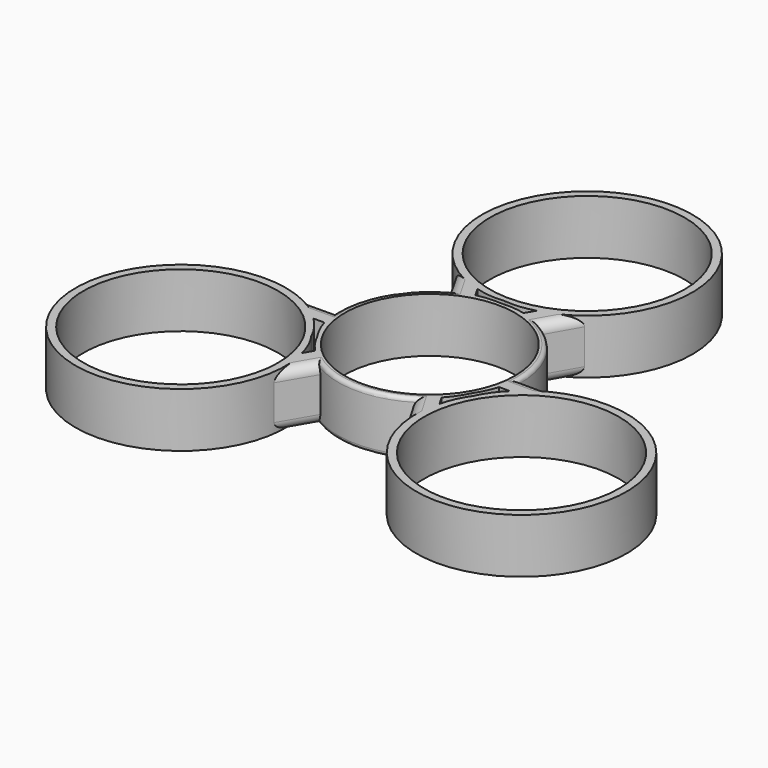
from build123d import *

# Parameters (mm, degrees)
F0_R     = 12.7
F0_R_2   = 11.1125
F1_DEPTH = 7.112
F2_R     = 1.27
F3_R     = 0.50799


# Not quite as in the source:
# - a fillet or chamfer is up to 0.001 mm smaller than in the source, because OpenCascade refuses the exact size
# - ends of sketch curves that miss each other by under 0.0002 mm in the source are joined


with BuildPart() as f1:
    # F0 (on Top) → F1 (new body)
    with BuildSketch(Plane.XY):
        with BuildLine():
            ThreePointArc((8.3638022209, 14.7734709329), (0, 39.3942033225), (-8.3638022209, 14.7734709329))
            Line((-8.3638022209, 14.7734709329), (-5.8662054787, 10.3931058657))
            ThreePointArc((-5.8662054787, 10.3931058657), (-10.3354618297, 5.9671806592), (-11.9337964262, -0.1162717145))
            Line((-11.9337964262, -0.1162717145), (-16.9761022194, -0.1434727603))
            ThreePointArc((-16.9761022194, -0.1434727603), (-34.1163779507, -19.6971066641), (-8.6122978741, -14.6300019249))
            Line((-8.6122978741, -14.6300019249), (-6.0675894575, -10.276836791))
            ThreePointArc((-6.0675894575, -10.276836791), (0, -11.934362834), (6.0675894575, -10.276836791))
            Line((6.0675894575, -10.276836791), (8.6122978741, -14.6300019249))
            ThreePointArc((8.6122978741, -14.6300019249), (34.1163779507, -19.6971066641), (16.9761022194, -0.1434727603))
            Line((16.9761022194, -0.1434727603), (11.9337964262, -0.1162717145))
            ThreePointArc((11.9337964262, -0.1162717145), (10.3354618297, 5.9671806592), (5.8662054787, 10.3931058657))
            Line((5.8662054787, 10.3931058657), (8.3638022209, 14.7734709329))
        make_face()
        with Locations((-22.225, -12.83160756)):
            Circle(F0_R, mode=Mode.SUBTRACT)
        with BuildLine():
            ThreePointArc((-8.9782080284, -9.6422017781), (-9.6052965229, -7.7965006784), (-10.5814479311, -6.109200777))
            ThreePointArc((-10.5814479311, -6.109200777), (-11.5546165578, -4.4201787661), (-12.8394961357, -2.9542534612))
            Line((-12.8394961357, -2.9542534612), (-11.4007424563, -2.9542534612))
            ThreePointArc((-11.4007424563, -2.9542534612), (-10.8372927454, -4.4313928826), (-10.042581953, -5.7980864121))
            ThreePointArc((-10.042581953, -5.7980864121), (-9.2563462346, -7.1696730271), (-8.258831006, -8.3962046475))
            Line((-8.258831006, -8.3962046475), (-8.9782080284, -9.6422017781))
        make_face(mode=Mode.SUBTRACT)
        with Locations((22.225, -12.83160756)):
            Circle(F0_R, mode=Mode.SUBTRACT)
        with BuildLine():
            Line((11.4007424563, -2.9542534612), (12.8394961357, -2.9542534612))
            ThreePointArc((12.8394961357, -2.9542534612), (11.5546165578, -4.4201787661), (10.5814479311, -6.109200777))
            ThreePointArc((10.5814479311, -6.109200777), (9.6052965229, -7.7965006784), (8.9782080284, -9.6422017781))
            Line((8.9782080284, -9.6422017781), (8.258831006, -8.3962046475))
            ThreePointArc((8.258831006, -8.3962046475), (9.2563462346, -7.1696730271), (10.042581953, -5.7980864121))
            ThreePointArc((10.042581953, -5.7980864121), (10.8372927454, -4.4313928826), (11.4007424563, -2.9542534612))
        make_face(mode=Mode.SUBTRACT)
        Circle(F0_R_2, mode=Mode.SUBTRACT)
        with BuildLine():
            ThreePointArc((-3.8612913684, 12.5964559897), (-1.9493229697, 12.2166805672), (-2.6876e-06, 12.2184031057))
            ThreePointArc((-2.6876e-06, 12.2184031057), (1.9493202828, 12.2166814247), (3.8612885145, 12.5964576884))
            Line((3.8612885145, 12.5964576884), (3.1419093526, 11.3504602412))
            ThreePointArc((3.1419093526, 11.3504602412), (1.5809467105, 11.6010677307), (0, 11.5961742969))
            ThreePointArc((0, 11.5961742969), (-1.5809492634, 11.6010670352), (-3.141914346, 11.350458859))
            Line((-3.141914346, 11.350458859), (-3.8612913684, 12.5964559897))
        make_face(mode=Mode.SUBTRACT)
        with Locations((0, 25.6632216382)):
            Circle(F0_R, mode=Mode.SUBTRACT)
    extrude(amount=F1_DEPTH)

    # F2
    f2_edges = [f1.edges().sort_by_distance(p)[0] for p in [
        (-7.339944, -12.453419, 7.112),
        (-14.454949, -0.129872, 7.112),
        (7.339944, -12.453419, 7.112),
        (14.454949, -0.129872, 7.112),
        (7.115004, 12.583288, 7.112),
        (-7.115004, 12.583288, 7.112),
        (-7.339944, -12.453419, 0),
        (7.339944, -12.453419, 0),
        (14.454949, -0.129872, 0),
        (7.115004, 12.583288, 0),
        (-7.115004, 12.583288, 0),
        (-14.454949, -0.129872, 0),
    ]]
    fillet(f2_edges, radius=F2_R)

    # F3 (radius 0.508 in the source; OpenCascade refuses exactly that, so slightly less here)
    f3_edges = [f1.edges().sort_by_distance(p)[0] for p in [
        (-10.335462, 5.967181, 7.112),
        (0, -11.934363, 7.112),
        (10.335462, 5.967181, 7.112),
        (10.335462, 5.967181, 0),
        (-10.335462, 5.967181, 0),
        (0, -11.934363, 0),
    ]]
    fillet(f3_edges, radius=F3_R)


solid = f1.part
